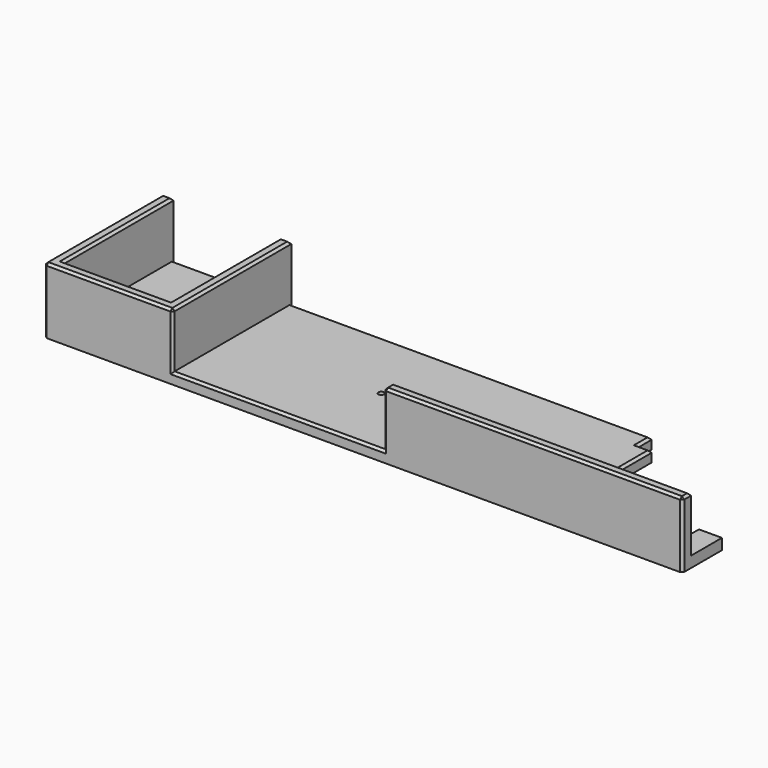
from build123d import *

# Parameters (mm, degrees)
F1_DEPTH  = 9.5
F2_W      = 9.5
F2_H      = 119.5
F2_H_2    = 9.5
F2_W_2    = 93
F3_DEPTH  = 48
F5_DEPTH  = 9.5
F6_R      = 2.5
F7_DEPTH  = 25.4
F8_W      = 15
F8_H      = 12.7057269514
F9_DEPTH  = 9.501
F10_W     = 260.0785551071
F10_H     = 9.5
F11_DEPTH = 48
F12_SIZE  = 2


# Not quite as in the source:
# - a feature names something its author has since deleted; it is built from what else it names


with BuildPart() as f1:
    # F0 (on Top) → F1 (new body)
    with BuildSketch(Plane.XY):
        Polygon((0, 129), (0, 0), (556, 0), (556, 43), (438, 43), (438, 114.0399202704), (426, 114.0399202704), (426, 33.5), (310, 33.5), (310, 83.1064879894), (302.5, 83.1064879894), (302.5, 129), align=None)
    extrude(amount=F1_DEPTH)

    # F2 (on face) → F3 (join)
    with BuildSketch(Plane.XY.offset(9.5)):
        with Locations((4.75, 69.25)):
            Rectangle(F2_W, F2_H)
        with Locations((4.75, 4.75)):
            Rectangle(F2_W, F2_H_2)
        with Locations((56, 4.75)):
            Rectangle(F2_W_2, F2_H_2)
        with Locations((107.25, 69.25)):
            Rectangle(F2_W, F2_H)
        with Locations((107.25, 4.75)):
            Rectangle(F2_W, F2_H_2)
    extrude(amount=F3_DEPTH)

    # F4 (on face) → F5 (join)
    with BuildSketch(Plane.XY.offset(9.5)):
        Polygon((426, 129), (302.5, 129), (302.5, 83.1064879894), (310, 83.1064879894), (310, 33.5), (426, 33.5), align=None)
    extrude(amount=-F5_DEPTH)

    # F6 (on face) → F7 (cut)
    with BuildSketch(Plane.XY.offset(9.5)):
        with BuildLine():
            ThreePointArc((244.5, 64.5), (242, 67), (239.5, 64.5))
            Line((239.5, 64.5), (244.5, 64.5))
        make_face()
        with BuildLine():
            Line((244.5, 64.5), (239.5, 64.5))
            ThreePointArc((239.5, 64.5), (242, 62), (244.5, 64.5))
        make_face()
        with Locations((376, 64.5)):
            Circle(F6_R)
    extrude(amount=-F7_DEPTH, mode=Mode.SUBTRACT)

    # F8 (on face) → F9 (cut, through all)
    with BuildSketch(Plane.XY.offset(9.5)):
        with Locations((463.5, 36.6471365243)):
            Rectangle(F8_W, F8_H)
        with Locations((528.5, 36.6471365243)):
            Rectangle(F8_W, F8_H)
    extrude(amount=-F9_DEPTH, mode=Mode.SUBTRACT)

    # F10 (on face) → F11 (join)
    with BuildSketch(Plane.XY.offset(9.5)):
        with Locations((425.9607224464, 4.75)):
            Rectangle(F10_W, F10_H)
    extrude(amount=F11_DEPTH)

    # F12
    f12_edges = [f1.edges().sort_by_distance(p)[0] for p in [
        (0, 64.5, 57.5),
        (9.5, 69.25, 57.5),
        (56, 0, 57.5),
        (56, 9.5, 57.5),
        (102.5, 69.25, 57.5),
        (112, 64.5, 57.5),
        (107.25, 129, 57.5),
        (4.75, 129, 57.5),
        (56, 129, 9.5),
        (269, 129, 9.5),
        (203.960722, 0, 9.5),
        (425.960722, 0, 57.5),
        (425.960722, 9.5, 57.5),
        (556, 4.75, 57.5),
        (438, 78.51996, 9.5),
        (426, 121.51996, 9.5),
        (432, 114.03992, 9.5),
        (112, 0, 33.5),
        (0, 0, 28.75),
        (295.921445, 4.75, 57.5),
        (295.921445, 0, 33.5),
        (556, 0, 28.75),
    ]]
    chamfer(f12_edges, length=F12_SIZE)


solid = f1.part
